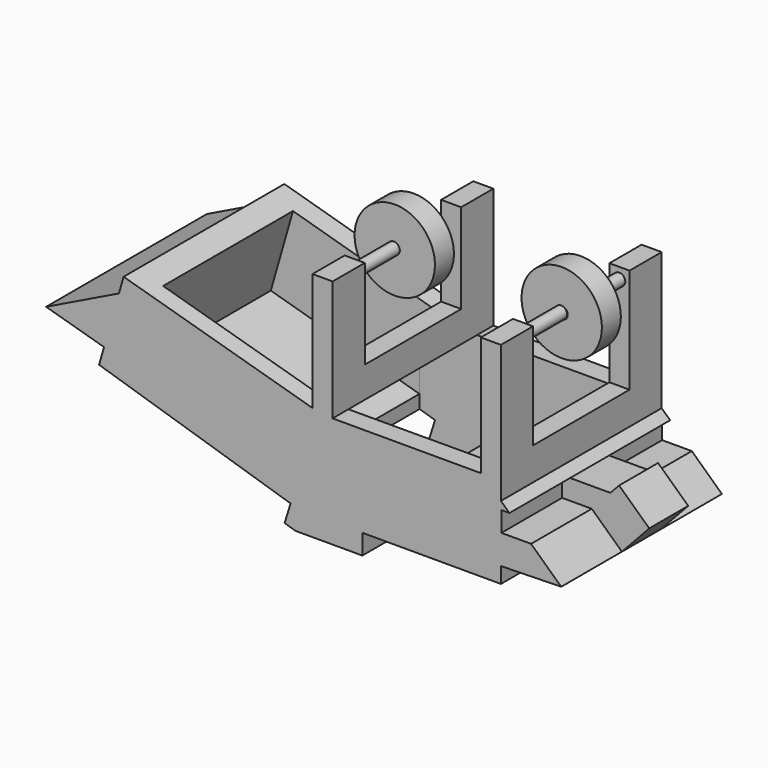
from build123d import *

# Parameters (mm, degrees)
F0_W      = 12.7
F0_H      = 75.5161463809
F1_DEPTH  = 127
F2_W      = 76.2
F2_H      = 66.2636627701
F3_DEPTH  = 25.4
F4_W      = 76.2
F4_H      = 56.6441606358
F5_DEPTH  = 25.4
F7_DEPTH  = 50.8
F8_W      = 91.44
F8_H      = 96.52
F9_DEPTH  = 50.8
F10_DEPTH = 50.8
F11_DEPTH = 25.4
F12_W     = 16.2214900825
F12_H     = 96.52
F13_DEPTH = 25.4
F14_W     = 107.6614900825
F14_H     = 4.7919526836
F15_DEPTH = 50.8
F16_W     = 107.6614900825
F16_H     = 1.27
F17_DEPTH = 50.8
F18_W     = 25.4
F18_H     = 101.6
F19_DEPTH = 50.8
F21_DEPTH = 50.8
F22_W     = 25.9920891664
F22_H     = 30.7906605303
F23_DEPTH = 50.8
F24_DEPTH = 43.18
F25_DEPTH = 25.4
F26_R     = 3.81
F27_DEPTH = 30.48
F28_R     = 3.81
F29_DEPTH = 30.48
F30_R     = 25.4
F30_R_2   = 3.81
F31_DEPTH = 14.986
F34_R     = 3.81
F35_DEPTH = 30.48
F36_R     = 25.4
F36_R_2   = 3.81
F37_DEPTH = 14.986


# Not quite as in the source:
# - the program builds the solid bodies; features that only make, move or delete a surface that nothing else refers to are left out


with BuildPart() as f1:
    # F0 (on Front) → F1 (new body)
    with BuildSketch(Plane.XZ):
        Polygon((-87.5999455111, 0), (0, 0), (0, 9.9594512863), (0, 46.2035047115), (0, 57.53631645), (-12.7, 57.53631645), (-106.3919453168, 57.53631645), (-113.4251185967, 57.53631645), (-119.0919453168, 59.1605978149), (-238.5092618621, 93.3891584363), (-241.4471621132, 83.1393507349), (-250.8809689206, 50.2264886893), (-254, 39.3447479744), (-132.9504583663, 1.5528194825), (-127.9766956054, 0), align=None)
        Polygon((-287.50616107, 60.7243599029), (-250.8809689206, 50.2264886893), (-241.4471621132, 83.1393507349), align=None)
        Polygon((-87.5999455111, -12.7), (-87.5999455111, 0), (-127.9766956054, 0), (-132.9504583663, 1.5528194825), (-136.7352611956, -10.5701037435), (-129.9130910692, -12.7), align=None)
        Polygon((-113.4251185967, 57.53631645), (-106.3919453168, 57.53631645), (-106.3919453168, 133.73631645), (-119.0919453168, 133.73631645), (-119.0919453168, 59.1605978149), align=None)
        with Locations((-6.35, 95.2943896404)):
            Rectangle(F0_W, F0_H)
        Polygon((43.4708868936, 41.215249927), (5.3708868936, 41.215249927), (19.0450608273, 28.515249927), (43.4708868936, 28.515249927), align=None)
        Polygon((0, 46.2035047115), (0, 9.9594512863), (38.0901216545, 10.8269951425), (19.0450608273, 28.515249927), (5.3708868936, 41.215249927), align=None)
    extrude(amount=-F1_DEPTH)

    # F2 (on face) → F3 (cut)
    with BuildSketch(Plane.YZ):
        with Locations((63.5, 99.9206314458)):
            Rectangle(F2_W, F2_H)
    extrude(amount=-F3_DEPTH, mode=Mode.SUBTRACT)

    # F4 (on face) → F5 (cut)
    with BuildSketch(Plane(origin=(-119.0919453168, 0, 0), x_dir=(0, -1, 0), z_dir=(-1, 0, 0))):
        with Locations((-63.5, 105.4142361321)):
            Rectangle(F4_W, F4_H)
    extrude(amount=-F5_DEPTH, mode=Mode.SUBTRACT)

    # F6 (on face) → F7 (cut)
    with BuildSketch(Plane.XY.offset(57.53631645)):
        Polygon((-20.7326539246, 114.0913581697), (-91.852224491, 114.0913581697), (-91.852224491, 12.4913581697), (-20.7326539246, 12.7385068121), align=None)
    extrude(amount=-F7_DEPTH, mode=Mode.SUBTRACT)

    # F8 (on face) → F9 (cut)
    with BuildSketch(Plane(origin=(6.6284267866, 0, 23.125393689), x_dir=(0.9612911325, 0, -0.2755346775), z_dir=(0.2755346775, 0, 0.9612911325))):
        with Locations((-192.7243173122, 64.3972861033)):
            Rectangle(F8_W, F8_H)
    extrude(amount=-F9_DEPTH, mode=Mode.SUBTRACT)

    # F10 (cut): a face of the model
    f10_faces = [f1.faces().sort_by_distance(p)[0] for p in [
        (-91.852224491, 63.2913581697, 32.13631645),
    ]]
    extrude(f10_faces, amount=-F10_DEPTH, mode=Mode.SUBTRACT)

    # F11 (cut): a face of the model
    f11_faces = [f1.faces().sort_by_distance(p)[0] for p in [
        (-145.6674529992, 64.3972861033, 25.3161834597),
    ]]
    extrude(f11_faces, amount=-F11_DEPTH, mode=Mode.SUBTRACT)

    # F12 (on face) → F13 (cut)
    with BuildSketch(Plane(origin=(6.6284267866, 0, 23.125393689), x_dir=(0.9612911325, 0, -0.2755346775), z_dir=(0.2755346775, 0, 0.9612911325))):
        with Locations((-138.893572271, 64.3972861033)):
            Rectangle(F12_W, F12_H)
    extrude(amount=-F13_DEPTH, mode=Mode.SUBTRACT)

    # F14 (on face) → F15 (cut)
    with BuildSketch(Plane(origin=(6.6284267866, 0, 23.125393689), x_dir=(0.9612911325, 0, -0.2755346775), z_dir=(0.2755346775, 0, 0.9612911325))):
        with Locations((-184.613572271, 13.7413097615)):
            Rectangle(F14_W, F14_H)
    extrude(amount=-F15_DEPTH, mode=Mode.SUBTRACT)

    # F16 (on face) → F17 (cut)
    with BuildSketch(Plane(origin=(6.6284267866, 0, 23.125393689), x_dir=(0.9612911325, 0, -0.2755346775), z_dir=(0.2755346775, 0, 0.9612911325))):
        with Locations((-184.613572271, 113.2922861033)):
            Rectangle(F16_W, F16_H)
    extrude(amount=-F17_DEPTH, mode=Mode.SUBTRACT)

    # F18 (on face) → F19 (cut)
    with BuildSketch(Plane.XY.offset(6.73631645)):
        with Locations((-129.952224491, 63.2913581697)):
            Rectangle(F18_W, F18_H)
    extrude(amount=-F19_DEPTH, mode=Mode.SUBTRACT)

    # F20 (on face) → F21 (cut)
    with BuildSketch(Plane.XY.offset(6.73631645)):
        Polygon((-117.252224491, 12.4913581697), (-104.552224491, 12.4913581697), (-91.852224491, 12.4913581697), (-92.2052961121, 114.0913581697), (-117.252224491, 114.0913581697), align=None)
    extrude(amount=-F21_DEPTH, mode=Mode.SUBTRACT)

    # F22 (on face) → F23 (join)
    with BuildSketch(Plane(origin=(23.0388020149, 0, 24.8060303918), x_dir=(0.7327252806, 0, -0.68052455), z_dir=(0.68052455, 0, 0.7327252806))):
        with Locations((7.5455144958, 63.3634831756)):
            Rectangle(F22_W, F22_H)
    extrude(amount=F23_DEPTH)

    # F24 (cut): faces of the model
    f24_faces = [f1.faces().sort_by_distance(p)[0] for p in [
        (43.4708868936, 23.9840764552, 34.865249927),
        (43.4708868936, 102.8794067204, 34.865249927),
    ]]
    extrude(f24_faces, amount=-F24_DEPTH, mode=Mode.SUBTRACT)

    # F25 (cut): a face of the model
    f25_faces = [f1.faces().sort_by_distance(p)[0] for p in [
        (63.1382383827, 63.3634831756, 56.8935667881),
    ]]
    extrude(f25_faces, amount=-F25_DEPTH, mode=Mode.SUBTRACT)

    # F26 (on face) → F27 (join)
    with BuildSketch(Plane.XZ.offset(-101.6)):
        with Locations((-6.4799388689, 126.0670712375)):
            Circle(F26_R)
    extrude(amount=F27_DEPTH)

    # F28 (on face) → F29 (join)
    with BuildSketch(Plane(origin=(0, 25.4, 0), x_dir=(-1, 0, 0), z_dir=(0, 1, 0))):
        with Locations((6.6545831251, 126.2898803812)):
            Circle(F28_R)
    extrude(amount=F29_DEPTH)

    # F34 (on face) → F35 (join)
    with BuildSketch(Plane(origin=(0, 25.4, 0), x_dir=(-1, 0, 0), z_dir=(0, 1, 0))):
        with Locations((112.426199019, 127.5002658367)):
            Circle(F34_R)
    extrude(amount=F35_DEPTH)


with BuildPart() as f31:
    # F30 (on face) → F31 (new body)
    with BuildSketch(Plane.XZ.offset(-71.12)):
        with Locations((-6.4799388689, 126.0670712375)):
            Circle(F30_R)
        with Locations((-6.4799388689, 126.0670712375)):
            Circle(F30_R_2, mode=Mode.SUBTRACT)
    extrude(amount=F31_DEPTH)


with BuildPart() as f37:
    # F36 (on face) → F37 (new body)
    with BuildSketch(Plane(origin=(0, 55.88, 0), x_dir=(-1, 0, 0), z_dir=(0, 1, 0))):
        with Locations((111.809797585, 126.7330497503)):
            Circle(F36_R)
        with Locations((112.426199019, 127.5002658367)):
            Circle(F36_R_2, mode=Mode.SUBTRACT)
    extrude(amount=F37_DEPTH)


solid = Compound([f1.part, f31.part, f37.part])
